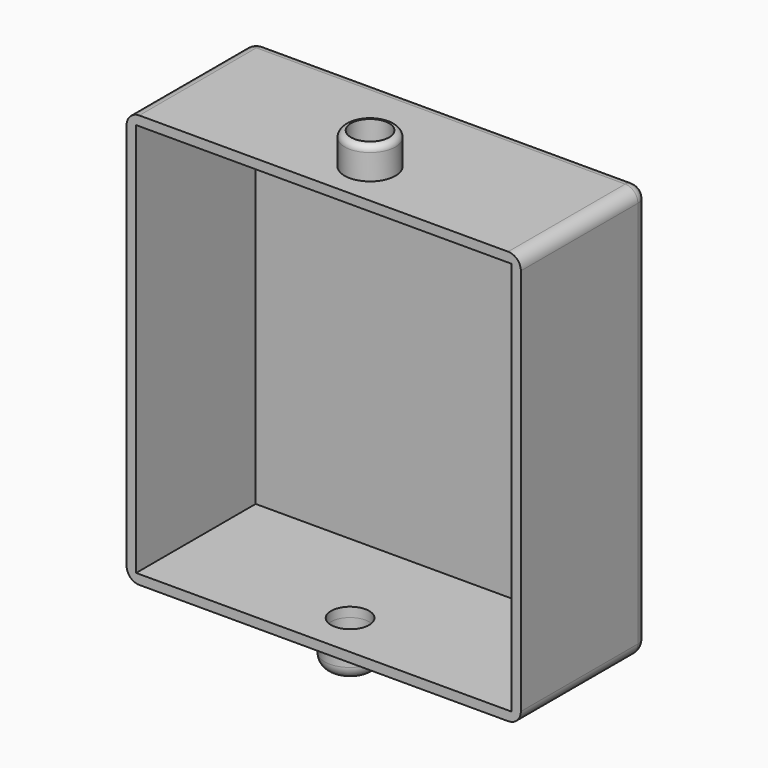
from build123d import *

# Parameters (mm, degrees)
F0_W     = 59
F0_H     = 62
F1_DEPTH = 1.5
F0_W_2   = 62
F0_H_2   = 65
F2_DEPTH = 25
F3_R     = 3
F4_DEPTH = 25
F3_R_2   = 4
F5_DEPTH = 5
F6_R     = 3
F7_DEPTH = 25
F6_R_2   = 4
F8_DEPTH = 5
F9_R     = 2
F10_R    = 0.99999


# Not quite as in the source:
# - a fillet or chamfer that OpenCascade refuses, or shapes differently, is made with other operations: its cross-section is extruded or revolved along the edge and cut away or added
# - a fillet or chamfer is up to 0.001 mm smaller than in the source, because OpenCascade refuses the exact size
# - a feature names something its author has since deleted; it is built from what else it names


with BuildPart() as f1:
    # F0 (on Front) → F1 (new body)
    with BuildSketch(Plane.XZ):
        with Locations((-27.9035090804, 32.3903523386)):
            Rectangle(F0_W, F0_H)
    extrude(amount=F1_DEPTH)

    # F0 (on Front) → F2 (join)
    with BuildSketch(Plane.XZ):
        with Locations((-27.9035090804, 32.3903523386)):
            Rectangle(F0_W_2, F0_H_2)
        with Locations((-27.9035090804, 32.3903523386)):
            Rectangle(F0_W, F0_H, mode=Mode.SUBTRACT)
    extrude(amount=F2_DEPTH)

    # F3 (on face) → F4 (cut)
    with BuildSketch(Plane(origin=(0, 0, -0.1096476614), x_dir=(1, 0, 0), z_dir=(0, 0, -1))):
        with Locations((-29.4035090804, 17.9373911147)):
            Circle(F3_R)
    extrude(amount=-F4_DEPTH, mode=Mode.SUBTRACT)

    # F3 (on face) → F5 (join)
    with BuildSketch(Plane(origin=(0, 0, -0.1096476614), x_dir=(1, 0, 0), z_dir=(0, 0, -1))):
        with Locations((-29.4035090804, 17.9373911147)):
            Circle(F3_R_2)
        with Locations((-29.4035090804, 17.9373911147)):
            Circle(F3_R, mode=Mode.SUBTRACT)
    extrude(amount=F5_DEPTH)

    # F6 (on face) → F7 (cut)
    with BuildSketch(Plane.XY.offset(64.8903523386)):
        with Locations((-26.3056773692, -17.8879302088)):
            Circle(F6_R)
    extrude(amount=-F7_DEPTH, mode=Mode.SUBTRACT)

    # F6 (on face) → F8 (join)
    with BuildSketch(Plane.XY.offset(64.8903523386)):
        with Locations((-26.3056773692, -17.8879302088)):
            Circle(F6_R_2)
        with Locations((-26.3056773692, -17.8879302088)):
            Circle(F6_R, mode=Mode.SUBTRACT)
    extrude(amount=F8_DEPTH)

    # F9
    f9_edges = [f1.edges().sort_by_distance(p)[0] for p in [
        (-58.903509, 0, 32.390352),
        (-58.903509, -12.5, -0.109648),
        (-58.903509, -12.5, 64.890352),
        (-27.903509, 0, -0.109648),
        (-27.903509, 0, 64.890352),
        (3.096491, -12.5, 64.890352),
        (3.096491, 0, 32.390352),
        (3.096491, -12.5, -0.109648),
    ]]
    fillet(f9_edges, radius=F9_R)

    # F10 (radius 1 in the source; OpenCascade refuses exactly that, so slightly less here)
    f10_edges = [f1.edges().sort_by_distance(p)[0] for p in [
        (-30.305677, -17.88793, 69.890352),
    ]]
    fillet(f10_edges, radius=F10_R)

    # F11: fillet of radius 2 on 1 edges, made by hand

    # F11_s1 → F11_t2 (revolve, cut)
    with BuildSketch(Plane.XZ.offset(17.9373911147)):
        with BuildLine():
            ThreePointArc((-25.4035090804, -3.3775968539), (-25.6714582728, -4.3775968539), (-26.4035090804, -5.1096476614))
            Line((-26.4035090804, -5.1096476614), (-25.4035090804, -5.1096476614))
            Line((-25.4035090804, -5.1096476614), (-25.4035090804, -3.3775968539))
        make_face()
    revolve(axis=Axis((-29.4035090804, -17.9373911147, -5.1096476614), (0, 0, -1)), mode=Mode.SUBTRACT)


with BuildPart() as f12_1:
    # F12: copy of F1
    add(f1.part)


with BuildPart() as f14_1:
    # F14: copy of F1
    add(f1.part)


solid = Compound([f1.part, f14_1.part])
